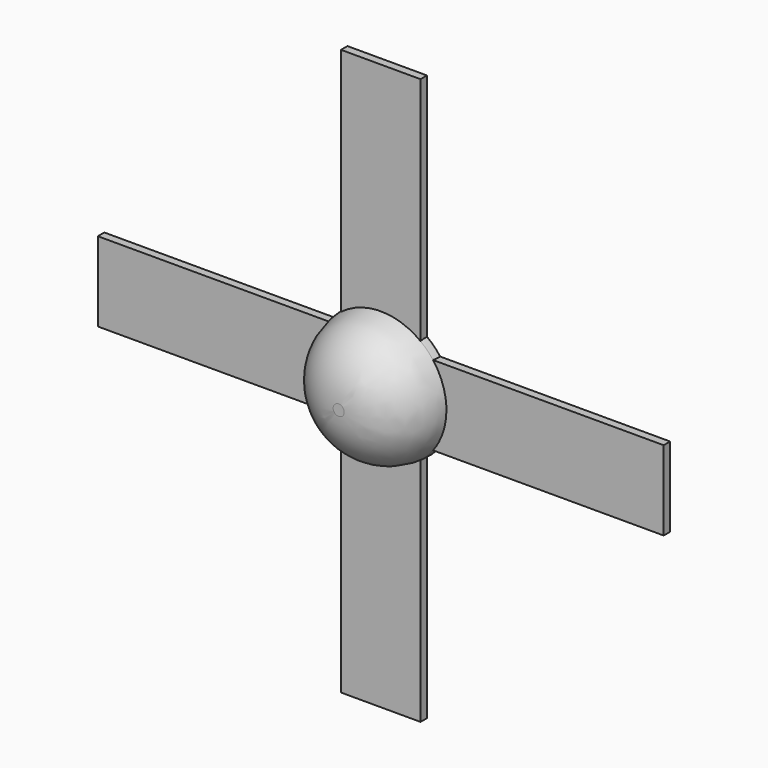
from build123d import *

# Parameters (mm, degrees)
F0_R     = 4.1575260002
F1_DEPTH = 3.81
F2_W     = 4.9914508127
F2_H     = 15.2679625899
F2_W_2   = 15.267963754
F2_H_2   = 4.9914494157
F3_DEPTH = 0.508


# Not quite as in the source:
# - a fillet or chamfer that OpenCascade refuses, or shapes differently, is made with other operations: its cross-section is extruded or revolved along the edge and cut away or added


with BuildPart() as f1:
    # F0 (on Front) → F1 (new body)
    with BuildSketch(Plane.XZ):
        Circle(F0_R)
    extrude(amount=F1_DEPTH)

    # F2 (on Front) → F3 (join)
    with BuildSketch(Plane.XZ):
        with Locations((0, 10.1297060028)):
            Rectangle(F2_W, F2_H)
        with Locations((-10.1297072833, 0)):
            Rectangle(F2_W_2, F2_H_2)
        Rectangle(F2_W, F2_H_2)
        with Locations((0, -10.1297060028)):
            Rectangle(F2_W, F2_H)
        with Locations((10.1297072833, 0)):
            Rectangle(F2_W_2, F2_H_2)
    extrude(amount=F3_DEPTH)

    # F4: fillet of radius 3.81 on 1 edges, made by hand


with BuildPart() as f4_tool2:
    # F4_s3 → F4_t4 (revolve)
    with BuildSketch(Plane.XY):
        with BuildLine():
            ThreePointArc((4.1575260002, 0), (3.0416028366, -2.6940768363), (0.3475260002, -3.81))
            Line((0.3475260002, -3.81), (4.1575260002, -3.81))
            Line((4.1575260002, -3.81), (4.1575260002, 0))
        make_face()
    revolve(axis=Axis((0, -3.81, 0), (0, -1, 0)))

    split(bisect_by=Plane.XZ.offset(0.508), keep=Keep.TOP)


with BuildPart() as f1_1:
    add(f1.part)

    # F4_t1: cut F4_tool2
    add(f4_tool2.part, mode=Mode.SUBTRACT)


with BuildPart() as f4_tool7:
    # F4_s8 → F4_t9 (revolve)
    with BuildSketch(Plane.XY):
        with BuildLine():
            ThreePointArc((4.1575260002, 0), (3.0416028366, -2.6940768363), (0.3475260002, -3.81))
            Line((0.3475260002, -3.81), (4.1575260002, -3.81))
            Line((4.1575260002, -3.81), (4.1575260002, 0))
        make_face()
    revolve(axis=Axis((0, -3.81, 0), (0, -1, 0)))

    split(bisect_by=Plane.XY.offset(2.4957247078), keep=Keep.TOP)

    split(bisect_by=Plane.YZ.offset(2.4957254063), keep=Keep.TOP)


with BuildPart() as f1_2:
    add(f1_1.part)

    # F4_t6: cut F4_tool7
    add(f4_tool7.part, mode=Mode.SUBTRACT)


with BuildPart() as f4_tool13:
    # F4_s14 → F4_t15 (revolve)
    with BuildSketch(Plane.XY):
        with BuildLine():
            ThreePointArc((4.1575260002, 0), (3.0416028366, -2.6940768363), (0.3475260002, -3.81))
            Line((0.3475260002, -3.81), (4.1575260002, -3.81))
            Line((4.1575260002, -3.81), (4.1575260002, 0))
        make_face()
    revolve(axis=Axis((0, -3.81, 0), (0, -1, 0)))

    split(bisect_by=Plane.XY.offset(-2.4957247078), keep=Keep.BOTTOM)

    split(bisect_by=Plane.YZ.offset(2.4957254063), keep=Keep.TOP)


with BuildPart() as f1_3:
    add(f1_2.part)

    # F4_t12: cut F4_tool13
    add(f4_tool13.part, mode=Mode.SUBTRACT)


with BuildPart() as f4_tool19:
    # F4_s20 → F4_t21 (revolve)
    with BuildSketch(Plane.XY):
        with BuildLine():
            ThreePointArc((4.1575260002, 0), (3.0416028366, -2.6940768363), (0.3475260002, -3.81))
            Line((0.3475260002, -3.81), (4.1575260002, -3.81))
            Line((4.1575260002, -3.81), (4.1575260002, 0))
        make_face()
    revolve(axis=Axis((0, -3.81, 0), (0, -1, 0)))

    split(bisect_by=Plane.XY.offset(2.4957247078), keep=Keep.TOP)

    split(bisect_by=Plane.YZ.offset(-2.4957254063), keep=Keep.BOTTOM)


with BuildPart() as f1_4:
    add(f1_3.part)

    # F4_t18: cut F4_tool19
    add(f4_tool19.part, mode=Mode.SUBTRACT)


with BuildPart() as f4_tool25:
    # F4_s26 → F4_t27 (revolve)
    with BuildSketch(Plane.XY):
        with BuildLine():
            ThreePointArc((4.1575260002, 0), (3.0416028366, -2.6940768363), (0.3475260002, -3.81))
            Line((0.3475260002, -3.81), (4.1575260002, -3.81))
            Line((4.1575260002, -3.81), (4.1575260002, 0))
        make_face()
    revolve(axis=Axis((0, -3.81, 0), (0, -1, 0)))

    split(bisect_by=Plane.XY.offset(-2.4957247078), keep=Keep.BOTTOM)

    split(bisect_by=Plane.YZ.offset(-2.4957254063), keep=Keep.BOTTOM)


with BuildPart() as f1_5:
    add(f1_4.part)

    # F4_t24: cut F4_tool25
    add(f4_tool25.part, mode=Mode.SUBTRACT)


solid = f1_5.part
